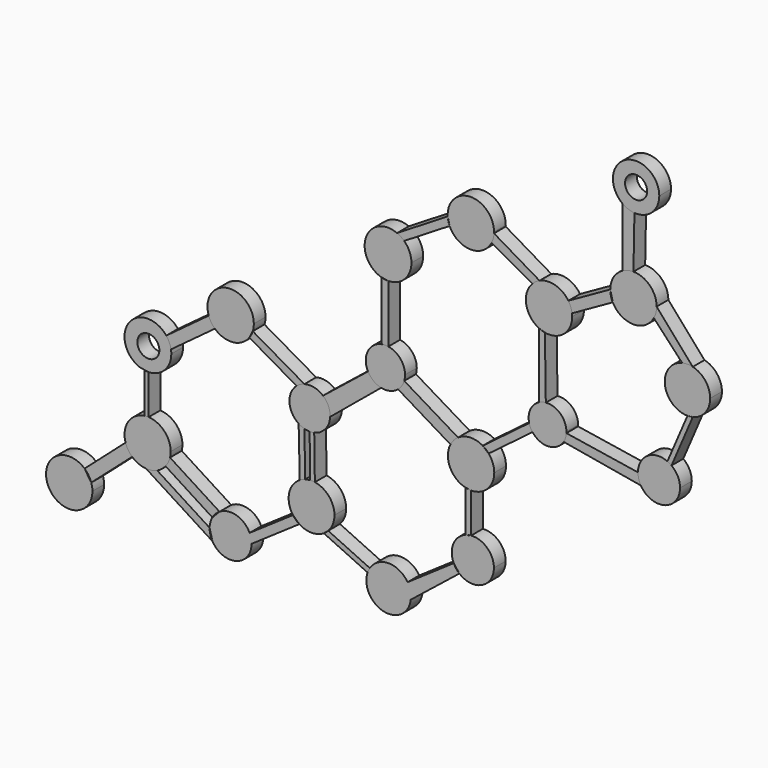
from build123d import *

# Parameters (mm, degrees)
F1_DEPTH = 2
F2_DEPTH = 2
F3_DEPTH = 2
F4_DEPTH = 2
F5_DEPTH = 2
F6_DEPTH = 2
F0_R     = 1.5066065713
F7_DEPTH = 2
F8_DEPTH = 2
F9_DEPTH = 2


# Not quite as in the source:
# - a feature names something its author has since deleted; it is built from what else it names


with BuildPart() as f1:
    # F0 (on Front) → F1 (new body)
    with BuildSketch(Plane.XZ):
        with BuildLine():
            ThreePointArc((-37.589425931, -3.0947996006), (-41.2739135306, 0.0261789427), (-43.7463731476, -4.1214588648))
            ThreePointArc((-43.7463731476, -4.1214588648), (-43.4052670506, -4.8209088), (-42.903755988, -5.4159468116))
            ThreePointArc((-42.903755988, -5.4159468116), (-40.446641178, -6.2439552219), (-38.1955916927, -4.9571812203))
            Line((-38.1955916927, -4.9571812203), (-37.7330076999, -4.0371317667))
            ThreePointArc((-37.7330076999, -4.0371317667), (-37.625527328, -3.5714036385), (-37.589425931, -3.0947996006))
        make_face()
        with BuildLine():
            Line((-43.7463731476, -4.1214588648), (-49.5391355238, -8.405172605))
            ThreePointArc((-49.5391355238, -8.405172605), (-49.1275958248, -9.0863151577), (-48.8971660779, -9.8480383571))
            Line((-48.8971660779, -9.8480383571), (-42.903755988, -5.4159468116))
            ThreePointArc((-42.903755988, -5.4159468116), (-43.4052670506, -4.8209088), (-43.7463731476, -4.1214588648))
        make_face()
    extrude(amount=F1_DEPTH)


with BuildPart() as f1b:
    # F0 (on Front) → F1, piece 2 (new body)
    with BuildSketch(Plane.XZ):
        with BuildLine():
            Line((-52.5149528088, -13.5454778642), (-52.5149528088, -19.0149929974))
            ThreePointArc((-52.5149528088, -19.0149929974), (-52.2351705303, -18.9893002665), (-51.9542118299, -18.9886305873))
            Line((-51.9542118299, -18.9886305873), (-51.9542118299, -13.5786520564))
            ThreePointArc((-51.9542118299, -13.5786520564), (-52.2353128072, -13.5744123442), (-52.5149528088, -13.5454778642))
        make_face()
    extrude(amount=F1_DEPTH)


with BuildPart() as f1c:
    # F0 (on Front) → F1, piece 3 (new body)
    with BuildSketch(Plane.XZ):
        with BuildLine():
            ThreePointArc((-60.6940817402, -28.0116869203), (-60.1449171731, -28.6432468808), (-59.7805504981, -29.396696701))
            Line((-59.7805504981, -29.396696701), (-54.1960356234, -24.4784262655))
            ThreePointArc((-54.1960356234, -24.4784262655), (-54.7415469087, -23.8352167765), (-55.0969163835, -23.0703549944))
            Line((-55.0969163835, -23.0703549944), (-60.6940817402, -28.0116869203))
        make_face()
    extrude(amount=F1_DEPTH)


with BuildPart() as f1d:
    # F0 (on Front) → F1, piece 4 (new body)
    with BuildSketch(Plane.XZ):
        with BuildLine():
            ThreePointArc((-60.6940817402, -28.0116869203), (-65.6698365107, -31.6876499309), (-59.622113901, -30.3853861988))
            ThreePointArc((-59.622113901, -30.3853861988), (-59.6619741252, -29.8847343541), (-59.7805504981, -29.396696701))
            Line((-59.7805504981, -29.396696701), (-60.6940817402, -28.0116869203))
        make_face()
    extrude(amount=F1_DEPTH)


with BuildPart() as f1e:
    # F0 (on Front) → F1, piece 5 (new body)
    with BuildSketch(Plane.XZ):
        with BuildLine():
            ThreePointArc((-49.0277410121, -22.8915968121), (-49.2667118253, -23.5421687766), (-49.6421238454, -24.124763615))
            Line((-49.6421238454, -24.124763615), (-43.2432128068, -28.2081848817))
            ThreePointArc((-43.2432128068, -28.2081848817), (-42.820009683, -27.6452432034), (-42.272247255, -27.2025688991))
            Line((-42.272247255, -27.2025688991), (-49.0277410121, -22.8915968121))
        make_face()
    extrude(amount=F1_DEPTH)


with BuildPart() as f1f:
    # F0 (on Front) → F1, piece 6 (new body)
    with BuildSketch(Plane.XZ):
        with BuildLine():
            ThreePointArc((-50.787159894, -25.0074364786), (-51.5279365519, -25.2380803723), (-52.3026155332, -25.2807317309))
            Line((-52.3026155332, -25.2807317309), (-43.2432128068, -31.0619275521))
            ThreePointArc((-43.2432128068, -31.0619275521), (-43.5341546393, -30.3463231537), (-43.623310519, -29.5789979072))
            Line((-43.623310519, -29.5789979072), (-50.787159894, -25.0074364786))
        make_face()
    extrude(amount=F1_DEPTH)


with BuildPart() as f1g:
    # F0 (on Front) → F1, piece 7 (new body)
    with BuildSketch(Plane.XZ):
        with BuildLine():
            ThreePointArc((-38.1675221321, -28.4145569119), (-37.9635998594, -29.0097260215), (-37.8945150633, -29.6350562169))
            Line((-37.8945150633, -29.6350562169), (-31.3852117273, -25.1609370351))
            ThreePointArc((-31.3852117273, -25.1609370351), (-31.85608698, -24.7950682197), (-32.2489724216, -24.3464876545))
            Line((-32.2489724216, -24.3464876545), (-38.1675221321, -28.4145569119))
        make_face()
        with BuildLine():
            Line((-43.623310519, -29.5789979072), (-43.2432128068, -31.0619275521))
            ThreePointArc((-43.2432128068, -31.0619275521), (-40.0208014314, -32.4029312754), (-37.8945150633, -29.6350562169))
            ThreePointArc((-37.8945150633, -29.6350562169), (-37.9635998594, -29.0097260215), (-38.1675221321, -28.4145569119))
            ThreePointArc((-38.1675221321, -28.4145569119), (-39.9479683628, -26.887644726), (-42.272247255, -27.2025688991))
            Line((-42.272247255, -27.2025688991), (-43.2432128068, -28.2081848817))
            ThreePointArc((-43.2432128068, -28.2081848817), (-43.5197045967, -28.8696225812), (-43.623310519, -29.5789979072))
        make_face()
    extrude(amount=F1_DEPTH)


with BuildPart() as f1h:
    # F0 (on Front) → F1, piece 8 (new body)
    with BuildSketch(Plane.XZ):
        with BuildLine():
            Line((-32.2489724216, -24.3464876545), (-31.3852117273, -25.1609370351))
            ThreePointArc((-31.3852117273, -25.1609370351), (-29.7102611512, -25.647195005), (-28.0353105751, -25.1609370351))
            Line((-28.0353105751, -25.1609370351), (-27.4344388987, -24.6650671828))
            ThreePointArc((-27.4344388987, -24.6650671828), (-26.8031946258, -23.6736847287), (-26.5823882584, -22.5193221122))
            ThreePointArc((-26.5823882584, -22.5193221122), (-27.3442929345, -20.4734034357), (-29.2588290055, -19.4241972599))
            ThreePointArc((-29.2588290055, -19.4241972599), (-29.5736466163, -19.3944340659), (-29.8898605352, -19.3966096864))
            ThreePointArc((-29.8898605352, -19.3966096864), (-30.2422535209, -19.4370221671), (-30.5878052461, -19.5170720902))
            ThreePointArc((-30.5878052461, -19.5170720902), (-30.9633331337, -19.6534192109), (-31.318418115, -19.8365213345))
            ThreePointArc((-31.318418115, -19.8365213345), (-32.7736054168, -21.8872534899), (-32.2489724216, -24.3464876545))
        make_face()
    extrude(amount=F1_DEPTH)


with BuildPart() as f1i:
    # F0 (on Front) → F1, piece 9 (new body)
    with BuildSketch(Plane.XZ):
        with BuildLine():
            ThreePointArc((-31.7558147602, -8.6673874945), (-32.7248214006, -10.9589087127), (-31.4725262417, -13.1087459619))
            ThreePointArc((-31.4725262417, -13.1087459619), (-31.0886843567, -13.3188508734), (-30.6766373042, -13.4661461312))
            ThreePointArc((-30.6766373042, -13.4661461312), (-30.3291581307, -13.5368601797), (-29.9755054116, -13.5627832774))
            ThreePointArc((-29.9755054116, -13.5627832774), (-29.6587887281, -13.5476755006), (-29.3458502966, -13.4966143551))
            ThreePointArc((-29.3458502966, -13.4966143551), (-28.9391104122, -13.3728908484), (-28.5559818149, -13.1886157349))
            Line((-28.5559818149, -13.1886157349), (-27.9344519304, -12.6986282105))
            ThreePointArc((-27.9344519304, -12.6986282105), (-27.3869776209, -11.8625662967), (-27.1704023319, -10.8869522401))
            ThreePointArc((-27.1704023319, -10.8869522401), (-27.1689132492, -10.8344270792), (-27.1684168293, -10.7818831599))
            ThreePointArc((-27.1684168293, -10.7818831599), (-27.4238049454, -9.6177281051), (-28.1430634561, -8.6673874945))
            ThreePointArc((-28.1430634561, -8.6673874945), (-29.3422205532, -8.0679615431), (-30.6824864397, -8.0992116323))
            ThreePointArc((-30.6824864397, -8.0992116323), (-31.2505437254, -8.3239955118), (-31.7558147602, -8.6673874945))
        make_face()
        with BuildLine():
            ThreePointArc((-37.7330076999, -4.0371317667), (-37.9266180846, -4.5161021168), (-38.1955916927, -4.9571812203))
            Line((-38.1955916927, -4.9571812203), (-31.7558147602, -8.6673874945))
            ThreePointArc((-31.7558147602, -8.6673874945), (-31.2505437254, -8.3239955118), (-30.6824864397, -8.0992116323))
            Line((-30.6824864397, -8.0992116323), (-37.7330076999, -4.0371317667))
        make_face()
        with BuildLine():
            Line((-22.0017600805, -3.7610865407), (-28.1430634561, -8.6673874945))
            ThreePointArc((-28.1430634561, -8.6673874945), (-27.4238049454, -9.6177281051), (-27.1684168293, -10.7818831599))
            ThreePointArc((-27.1684168293, -10.7818831599), (-27.1689132492, -10.8344270792), (-27.1704023319, -10.8869522401))
            Line((-27.1704023319, -10.8869522401), (-20.2051144084, -5.1334624074))
            ThreePointArc((-20.2051144084, -5.1334624074), (-21.2551436396, -4.6458808799), (-22.0017600805, -3.7610865407))
        make_face()
    extrude(amount=F1_DEPTH)


with BuildPart() as f1j:
    # F0 (on Front) → F1, piece 10 (new body)
    with BuildSketch(Plane.XZ):
        with BuildLine():
            ThreePointArc((-27.4344388987, -24.6650671828), (-27.7193761185, -24.931782603), (-28.0353105751, -25.1609370351))
            Line((-28.0353105751, -25.1609370351), (-22.0636666599, -27.9388750239))
            ThreePointArc((-22.0636666599, -27.9388750239), (-21.9298236713, -27.6131643375), (-21.7592310354, -27.3051066328))
            Line((-21.7592310354, -27.3051066328), (-27.4344388987, -24.6650671828))
        make_face()
    extrude(amount=F1_DEPTH)


with BuildPart() as f1k:
    # F0 (on Front) → F1, piece 11 (new body)
    with BuildSketch(Plane.XZ):
        with BuildLine():
            Line((-21.7592310354, -27.3051066328), (-22.0636666599, -27.9388750239))
            ThreePointArc((-22.0636666599, -27.9388750239), (-19.8661488676, -31.8951145091), (-16.1677066638, -29.2869656299))
            ThreePointArc((-16.1677066638, -29.2869656299), (-16.151956576, -29.1088509796), (-16.1467004913, -28.9301185889))
            ThreePointArc((-16.1467004913, -28.9301185889), (-16.2635315956, -28.0952311668), (-16.605049435, -27.324483426))
            ThreePointArc((-16.605049435, -27.324483426), (-19.1767786565, -25.8886276397), (-21.7592310354, -27.3051066328))
        make_face()
        with BuildLine():
            ThreePointArc((-16.1467004913, -28.9301185889), (-16.151956576, -29.1088509796), (-16.1677066638, -29.2869656299))
            Line((-16.1677066638, -29.2869656299), (-9.5345514551, -23.9877231505))
            ThreePointArc((-9.5345514551, -23.9877231505), (-9.97366221, -23.5326555023), (-10.3027902397, -22.9926744291))
            Line((-10.3027902397, -22.9926744291), (-16.605049435, -27.324483426))
            ThreePointArc((-16.605049435, -27.324483426), (-16.2635315956, -28.0952311668), (-16.1467004913, -28.9301185889))
        make_face()
    extrude(amount=F1_DEPTH)


with BuildPart() as f1l:
    # F0 (on Front) → F1, piece 12 (new body)
    with BuildSketch(Plane.XZ):
        with BuildLine():
            Line((-10.3027902397, -22.9926744291), (-9.5345514551, -23.9877231505))
            ThreePointArc((-9.5345514551, -23.9877231505), (-6.4727183358, -24.3792083426), (-4.8174418628, -21.7738019436))
            ThreePointArc((-4.8174418628, -21.7738019436), (-5.746709679, -19.6559016499), (-7.934436367, -18.9056401844))
            Line((-7.934436367, -18.9056401844), (-8.7257380015, -19.0864037696))
            ThreePointArc((-8.7257380015, -19.0864037696), (-10.3643389956, -20.6963441185), (-10.3027902397, -22.9926744291))
        make_face()
    extrude(amount=F1_DEPTH)


with BuildPart() as f1m:
    # F0 (on Front) → F1, piece 13 (new body)
    with BuildSketch(Plane.XZ):
        with BuildLine():
            Line((-8.7257380015, -13.3813622687), (-8.7257380015, -19.0864037696))
            ThreePointArc((-8.7257380015, -19.0864037696), (-8.3364915934, -18.9679863559), (-7.934436367, -18.9056401844))
            Line((-7.934436367, -18.9056401844), (-7.934436367, -13.4819080304))
            ThreePointArc((-7.934436367, -13.4819080304), (-8.3332683263, -13.4566709426), (-8.7257380015, -13.3813622687))
        make_face()
    extrude(amount=F1_DEPTH)


with BuildPart() as f1n:
    # F0 (on Front) → F1, piece 14 (new body)
    with BuildSketch(Plane.XZ):
        with BuildLine():
            ThreePointArc((-10.7471404399, -8.8686872464), (-10.8220432047, -11.6113089525), (-8.7257380015, -13.3813622687))
            Line((-8.7257380015, -13.3813622687), (-7.934436367, -13.4819080304))
            ThreePointArc((-7.934436367, -13.4819080304), (-5.6971007662, -12.555173281), (-4.7703660167, -10.3178376801))
            ThreePointArc((-4.7703660167, -10.3178376801), (-4.9665243966, -9.2210971833), (-5.5306776307, -8.2603428153))
            Line((-5.5306776307, -8.2603428153), (-6.3343212789, -7.5881906542))
            ThreePointArc((-6.3343212789, -7.5881906542), (-8.0398552645, -7.1555239643), (-9.7127880414, -7.7008152301))
            ThreePointArc((-9.7127880414, -7.7008152301), (-10.3030708851, -8.2200026768), (-10.7471404399, -8.8686872464))
        make_face()
    extrude(amount=F1_DEPTH)


with BuildPart() as f1o:
    # F0 (on Front) → F1, piece 15 (new body)
    with BuildSketch(Plane.XZ):
        with BuildLine():
            ThreePointArc((-6.3343212789, -7.5881906542), (-5.9044859902, -7.8907730644), (-5.5306776307, -8.2603428153))
            Line((-5.5306776307, -8.2603428153), (0.4520227905, -3.7452711915))
            ThreePointArc((0.4520227905, -3.7452711915), (0.1782258717, -3.2995528654), (0, -2.8077550232))
            Line((0, -2.8077550232), (-6.3343212789, -7.5881906542))
        make_face()
    extrude(amount=F1_DEPTH)


with BuildPart() as f1p:
    # F0 (on Front) → F1, piece 16 (new body)
    with BuildSketch(Plane.XZ):
        with BuildLine():
            Line((1.3706875539, 9.0120735989), (1.3706875539, 0.1384634004))
            ThreePointArc((1.3706875539, 0.1384634004), (1.8070578609, 0.3042996673), (2.2661741655, 0.3887563488))
            Line((2.2661741655, 0.3887563488), (2.1411547442, 8.7673323703))
            ThreePointArc((2.1411547442, 8.7673323703), (1.7480727228, 8.8649954394), (1.3706875539, 9.0120735989))
        make_face()
    extrude(amount=F1_DEPTH)


with BuildPart() as f1q:
    # F0 (on Front) → F1, piece 17 (new body)
    with BuildSketch(Plane.XZ):
        with BuildLine():
            ThreePointArc((0.4265353279, 14.0749963178), (-0.404465595, 11.3005324176), (1.3706875539, 9.0120735989))
            Line((1.3706875539, 9.0120735989), (2.1411547442, 8.7673323703))
            ThreePointArc((2.1411547442, 8.7673323703), (4.733812042, 9.4517433605), (5.8700526231, 11.8805800386))
            ThreePointArc((5.8700526231, 11.8805800386), (5.8634796502, 12.0844218734), (5.8437880405, 12.2874167948))
            ThreePointArc((5.8437880405, 12.2874167948), (5.6697146463, 12.9885654176), (5.3411360451, 13.6319525799))
            ThreePointArc((5.3411360451, 13.6319525799), (3.5849253378, 14.9201195219), (1.4122471164, 14.7680686579))
            ThreePointArc((1.4122471164, 14.7680686579), (0.8860935676, 14.46888958), (0.4265353279, 14.0749963178))
        make_face()
        with BuildLine():
            Line((11.0647150097, 16.8480308272), (5.3411360451, 13.6319525799))
            ThreePointArc((5.3411360451, 13.6319525799), (5.6697146463, 12.9885654176), (5.8437880405, 12.2874167948))
            Line((5.8437880405, 12.2874167948), (11.4082876159, 15.4141083547))
            ThreePointArc((11.4082876159, 15.4141083547), (11.1518067717, 16.1107764964), (11.0647150097, 16.8480308272))
        make_face()
    extrude(amount=F1_DEPTH)


with BuildPart() as f1r:
    # F0 (on Front) → F1, piece 18 (new body)
    with BuildSketch(Plane.XZ):
        with BuildLine():
            Line((-11.1217205665, 18.411016596), (-18.0350023015, 14.1660333875))
            ThreePointArc((-18.0350023015, 14.1660333875), (-17.5227173446, 13.8942737957), (-17.0679941499, 13.5343905243))
            Line((-17.0679941499, 13.5343905243), (-10.8623128482, 17.3448837072))
            ThreePointArc((-10.8623128482, 17.3448837072), (-11.0385836531, 17.8666196456), (-11.1217205665, 18.411016596))
        make_face()
        with BuildLine():
            Line((-20.166905726, 8.1530077233), (-19.2310512637, 8.0247410256))
            ThreePointArc((-19.2310512637, 8.0247410256), (-16.9970643361, 8.9740556334), (-16.074991523, 11.2194236533))
            ThreePointArc((-16.074991523, 11.2194236533), (-16.3337181015, 12.4789003135), (-17.0679941499, 13.5343905243))
            ThreePointArc((-17.0679941499, 13.5343905243), (-17.5227173446, 13.8942737957), (-18.0350023015, 14.1660333875))
            ThreePointArc((-18.0350023015, 14.1660333875), (-22.2811669762, 12.2870572206), (-20.166905726, 8.1530077233))
        make_face()
    extrude(amount=F1_DEPTH)


with BuildPart() as f1s:
    # F0 (on Front) → F1, piece 19 (new body)
    with BuildSketch(Plane.XZ):
        with BuildLine():
            Line((-20.166905726, 0.137046408), (-19.8017352531, 0.1608339565))
            ThreePointArc((-19.8017352531, 0.1608339565), (-19.5157580784, 0.1641787021), (-19.2310512637, 0.137046408))
            Line((-19.2310512637, 0.137046408), (-19.2310512637, 8.0247410256))
            ThreePointArc((-19.2310512637, 8.0247410256), (-19.7037450657, 8.0540967063), (-20.166905726, 8.1530077233))
            Line((-20.166905726, 8.1530077233), (-20.166905726, 0.137046408))
        make_face()
    extrude(amount=F1_DEPTH)


with BuildPart() as f1t:
    # F0 (on Front) → F1, piece 20 (new body)
    with BuildSketch(Plane.XZ):
        with BuildLine():
            Line((12.7010902051, 27.7389005383), (12.7010902051, 19.6188589877))
            ThreePointArc((12.7010902051, 19.6188589877), (13.4400376332, 19.9122139491), (14.22878536, 20.0121011774))
            Line((14.22878536, 20.0121011774), (14.3635529463, 27.1199137658))
            ThreePointArc((14.3635529463, 27.1199137658), (13.4880542027, 27.3105146948), (12.7010902051, 27.7389005383))
        make_face()
    extrude(amount=F1_DEPTH)


with BuildPart() as f1u:
    # F0 (on Front) → F1, piece 21 (new body)
    with BuildSketch(Plane.XZ):
        with BuildLine():
            Line((17.0147604727, 15.3481362132), (20.8823093018, 11.2153642881))
            ThreePointArc((20.8823093018, 11.2153642881), (21.6048193009, 11.3007129197), (22.3273293, 11.2153642881))
            Line((22.3273293, 11.2153642881), (17.3928557103, 16.8480308272))
            ThreePointArc((17.3928557103, 16.8480308272), (17.2968761696, 16.0746228071), (17.0147604727, 15.3481362132))
        make_face()
    extrude(amount=F1_DEPTH)


with BuildPart() as f1v:
    # F0 (on Front) → F1, piece 22 (new body)
    with BuildSketch(Plane.XZ):
        with BuildLine():
            Line((21.6048193009, 5.0990307341), (18.8674234688, -1.2655284067))
            ThreePointArc((18.8674234688, -1.2655284067), (19.1558508738, -1.4112828883), (19.4260827802, -1.5885100127))
            Line((19.4260827802, -1.5885100127), (22.3273293, 5.1843793656))
            ThreePointArc((22.3273293, 5.1843793656), (21.9685860832, 5.1204418129), (21.6048193009, 5.0990307341))
        make_face()
    extrude(amount=F1_DEPTH)


with BuildPart() as f1w:
    # F0 (on Front) → F1, piece 23 (new body)
    with BuildSketch(Plane.XZ):
        with BuildLine():
            ThreePointArc((5.073574541, -2.3652681739), (4.9561703, -2.9698845171), (4.6987535943, -3.5294212164))
            Line((4.6987535943, -3.5294212164), (15.2385687415, -5.3491116368))
            ThreePointArc((15.2385687415, -5.3491116368), (14.9453544153, -4.6498799144), (14.8452927694, -3.8982900596))
            Line((14.8452927694, -3.8982900596), (5.073574541, -2.3652681739))
        make_face()
    extrude(amount=F1_DEPTH)


with BuildPart() as f2:
    # F0 (on Front) → F2 (new body)
    with BuildSketch(Plane.XZ):
        with BuildLine():
            Line((-17.9006594395, -4.5664300135), (-10.7471404399, -8.8686872464))
            ThreePointArc((-10.7471404399, -8.8686872464), (-10.3030708851, -8.2200026768), (-9.7127880414, -7.7008152301))
            Line((-9.7127880414, -7.7008152301), (-17.0583318909, -3.2830707385))
            ThreePointArc((-17.0583318909, -3.2830707385), (-17.3856953146, -3.9863158479), (-17.9006594395, -4.5664300135))
        make_face()
    extrude(amount=F2_DEPTH)


with BuildPart() as f3:
    # F0 (on Front) → F3 (new body)
    with BuildSketch(Plane.XZ):
        with BuildLine():
            Line((-22.0017600805, -3.7610865407), (-28.1430634561, -8.6673874945))
            ThreePointArc((-28.1430634561, -8.6673874945), (-27.4238049454, -9.6177281051), (-27.1684168293, -10.7818831599))
            ThreePointArc((-27.1684168293, -10.7818831599), (-27.1689132492, -10.8344270792), (-27.1704023319, -10.8869522401))
            Line((-27.1704023319, -10.8869522401), (-20.2051144084, -5.1334624074))
            ThreePointArc((-20.2051144084, -5.1334624074), (-21.2551436396, -4.6458808799), (-22.0017600805, -3.7610865407))
        make_face()
    extrude(amount=F3_DEPTH)


with BuildPart() as f4:
    # F0 (on Front) → F4 (new body)
    with BuildSketch(Plane.XZ):
        with BuildLine():
            Line((-31.4725262417, -13.1087459619), (-31.318418115, -19.8365213345))
            ThreePointArc((-31.318418115, -19.8365213345), (-30.9633331337, -19.6534192109), (-30.5878052461, -19.5170720902))
            Line((-30.5878052461, -19.5170720902), (-30.6766373042, -13.4661461312))
            ThreePointArc((-30.6766373042, -13.4661461312), (-31.0886843567, -13.3188508734), (-31.4725262417, -13.1087459619))
        make_face()
    extrude(amount=F4_DEPTH)


with BuildPart() as f5:
    # F0 (on Front) → F5 (new body)
    with BuildSketch(Plane.XZ):
        with BuildLine():
            Line((-22.0017600805, -3.7610865407), (-28.1430634561, -8.6673874945))
            ThreePointArc((-28.1430634561, -8.6673874945), (-27.4238049454, -9.6177281051), (-27.1684168293, -10.7818831599))
            ThreePointArc((-27.1684168293, -10.7818831599), (-27.1689132492, -10.8344270792), (-27.1704023319, -10.8869522401))
            Line((-27.1704023319, -10.8869522401), (-20.2051144084, -5.1334624074))
            ThreePointArc((-20.2051144084, -5.1334624074), (-21.2551436396, -4.6458808799), (-22.0017600805, -3.7610865407))
        make_face()
    extrude(amount=F5_DEPTH)


with BuildPart() as f5b:
    # F0 (on Front) → F5, piece 2 (new body)
    with BuildSketch(Plane.XZ):
        with BuildLine():
            Line((-29.9755054116, -13.5627832774), (-29.8898605352, -19.3966096864))
            ThreePointArc((-29.8898605352, -19.3966096864), (-29.5736466163, -19.3944340659), (-29.2588290055, -19.4241972599))
            Line((-29.2588290055, -19.4241972599), (-29.3458502966, -13.4966143551))
            ThreePointArc((-29.3458502966, -13.4966143551), (-29.6587887281, -13.5476755006), (-29.9755054116, -13.5627832774))
        make_face()
    extrude(amount=F5_DEPTH)


with BuildPart() as f6:
    # F0 (on Front) → F6 (new body)
    with BuildSketch(Plane.XZ):
        with BuildLine():
            ThreePointArc((-37.589425931, -3.0947996006), (-41.2739135306, 0.0261789427), (-43.7463731476, -4.1214588648))
            ThreePointArc((-43.7463731476, -4.1214588648), (-43.4052670506, -4.8209088), (-42.903755988, -5.4159468116))
            ThreePointArc((-42.903755988, -5.4159468116), (-40.446641178, -6.2439552219), (-38.1955916927, -4.9571812203))
            Line((-38.1955916927, -4.9571812203), (-37.7330076999, -4.0371317667))
            ThreePointArc((-37.7330076999, -4.0371317667), (-37.625527328, -3.5714036385), (-37.589425931, -3.0947996006))
        make_face()
    extrude(amount=F6_DEPTH)


with BuildPart() as f6b:
    # F0 (on Front) → F6, piece 2 (new body)
    with BuildSketch(Plane.XZ):
        with BuildLine():
            Line((-52.5149528088, -13.4941877539), (-51.9542118299, -13.5786520564))
            ThreePointArc((-51.9542118299, -13.5786520564), (-49.7550373735, -12.6113053664), (-48.8517080577, -10.3850699666))
            ThreePointArc((-48.8517080577, -10.3850699666), (-48.863092847, -10.1155939096), (-48.8971660779, -9.8480383571))
            ThreePointArc((-48.8971660779, -9.8480383571), (-49.1275958248, -9.0863151577), (-49.5391355238, -8.405172605))
            ThreePointArc((-49.5391355238, -8.405172605), (-54.6558064246, -8.5412451571), (-53.0756937878, -13.4097234514))
            Line((-53.0756937878, -13.4097234514), (-52.5149528088, -13.4941877539))
        make_face()
        with Locations((-51.9861578941, -10.463591665)):
            Circle(F0_R, mode=Mode.SUBTRACT)
    extrude(amount=F6_DEPTH)


with BuildPart() as f6c:
    # F0 (on Front) → F6, piece 3 (new body)
    with BuildSketch(Plane.XZ):
        with BuildLine():
            ThreePointArc((-31.7558147602, -8.6673874945), (-32.7248214006, -10.9589087127), (-31.4725262417, -13.1087459619))
            ThreePointArc((-31.4725262417, -13.1087459619), (-31.0886843567, -13.3188508734), (-30.6766373042, -13.4661461312))
            ThreePointArc((-30.6766373042, -13.4661461312), (-30.3291581307, -13.5368601797), (-29.9755054116, -13.5627832774))
            ThreePointArc((-29.9755054116, -13.5627832774), (-29.6587887281, -13.5476755006), (-29.3458502966, -13.4966143551))
            ThreePointArc((-29.3458502966, -13.4966143551), (-28.9391104122, -13.3728908484), (-28.5559818149, -13.1886157349))
            Line((-28.5559818149, -13.1886157349), (-27.9344519304, -12.6986282105))
            ThreePointArc((-27.9344519304, -12.6986282105), (-27.3869776209, -11.8625662967), (-27.1704023319, -10.8869522401))
            ThreePointArc((-27.1704023319, -10.8869522401), (-27.1689132492, -10.8344270792), (-27.1684168293, -10.7818831599))
            ThreePointArc((-27.1684168293, -10.7818831599), (-27.4238049454, -9.6177281051), (-28.1430634561, -8.6673874945))
            ThreePointArc((-28.1430634561, -8.6673874945), (-29.3422205532, -8.0679615431), (-30.6824864397, -8.0992116323))
            ThreePointArc((-30.6824864397, -8.0992116323), (-31.2505437254, -8.3239955118), (-31.7558147602, -8.6673874945))
        make_face()
        with BuildLine():
            Line((-22.0017600805, -3.7610865407), (-28.1430634561, -8.6673874945))
            ThreePointArc((-28.1430634561, -8.6673874945), (-27.4238049454, -9.6177281051), (-27.1684168293, -10.7818831599))
            ThreePointArc((-27.1684168293, -10.7818831599), (-27.1689132492, -10.8344270792), (-27.1704023319, -10.8869522401))
            Line((-27.1704023319, -10.8869522401), (-20.2051144084, -5.1334624074))
            ThreePointArc((-20.2051144084, -5.1334624074), (-21.2551436396, -4.6458808799), (-22.0017600805, -3.7610865407))
        make_face()
    extrude(amount=F6_DEPTH)


with BuildPart() as f6d:
    # F0 (on Front) → F6, piece 4 (new body)
    with BuildSketch(Plane.XZ):
        with BuildLine():
            Line((-20.166905726, 8.1530077233), (-19.2310512637, 8.0247410256))
            ThreePointArc((-19.2310512637, 8.0247410256), (-16.9970643361, 8.9740556334), (-16.074991523, 11.2194236533))
            ThreePointArc((-16.074991523, 11.2194236533), (-16.3337181015, 12.4789003135), (-17.0679941499, 13.5343905243))
            ThreePointArc((-17.0679941499, 13.5343905243), (-17.5227173446, 13.8942737957), (-18.0350023015, 14.1660333875))
            ThreePointArc((-18.0350023015, 14.1660333875), (-22.2811669762, 12.2870572206), (-20.166905726, 8.1530077233))
        make_face()
    extrude(amount=F6_DEPTH)


with BuildPart() as f6e:
    # F0 (on Front) → F6, piece 5 (new body)
    with BuildSketch(Plane.XZ):
        with BuildLine():
            ThreePointArc((-4.8001403762, 18.614665292), (-8.0660878972, 21.7770950894), (-11.1217205665, 18.411016596))
            Line((-11.1217205665, 18.411016596), (-10.8623128482, 17.3448837072))
            ThreePointArc((-10.8623128482, 17.3448837072), (-8.0490426257, 15.4517323603), (-5.1383388486, 17.1913630363))
            ThreePointArc((-5.1383388486, 17.1913630363), (-4.9083346697, 17.7943222496), (-4.8054518647, 18.4314069094))
            ThreePointArc((-4.8054518647, 18.4314069094), (-4.8014685271, 18.5229976223), (-4.8001403762, 18.614665292))
        make_face()
    extrude(amount=F6_DEPTH)


with BuildPart() as f6f:
    # F0 (on Front) → F6, piece 6 (new body)
    with BuildSketch(Plane.XZ):
        with BuildLine():
            ThreePointArc((0, -2.8077550232), (0.1782258717, -3.2995528654), (0.4520227905, -3.7452711915))
            ThreePointArc((0.4520227905, -3.7452711915), (2.6322031678, -4.7551499279), (4.6987535943, -3.5294212164))
            ThreePointArc((4.6987535943, -3.5294212164), (4.9561703, -2.9698845171), (5.073574541, -2.3652681739))
            ThreePointArc((5.073574541, -2.3652681739), (5.07859903, -2.2724391904), (5.0802745854, -2.1794894287))
            ThreePointArc((5.0802745854, -2.1794894287), (4.2397953639, -0.2745584885), (2.2661741655, 0.3887563488))
            ThreePointArc((2.2661741655, 0.3887563488), (1.8070578609, 0.3042996673), (1.3706875539, 0.1384634004))
            ThreePointArc((1.3706875539, 0.1384634004), (0.1629760262, -1.0916214081), (0, -2.8077550232))
        make_face()
    extrude(amount=F6_DEPTH)


with BuildPart() as f6g:
    # F0 (on Front) → F6, piece 7 (new body)
    with BuildSketch(Plane.XZ):
        with BuildLine():
            ThreePointArc((0.4265353279, 14.0749963178), (-0.404465595, 11.3005324176), (1.3706875539, 9.0120735989))
            Line((1.3706875539, 9.0120735989), (2.1411547442, 8.7673323703))
            ThreePointArc((2.1411547442, 8.7673323703), (4.733812042, 9.4517433605), (5.8700526231, 11.8805800386))
            ThreePointArc((5.8700526231, 11.8805800386), (5.8634796502, 12.0844218734), (5.8437880405, 12.2874167948))
            ThreePointArc((5.8437880405, 12.2874167948), (5.6697146463, 12.9885654176), (5.3411360451, 13.6319525799))
            ThreePointArc((5.3411360451, 13.6319525799), (3.5849253378, 14.9201195219), (1.4122471164, 14.7680686579))
            ThreePointArc((1.4122471164, 14.7680686579), (0.8860935676, 14.46888958), (0.4265353279, 14.0749963178))
        make_face()
    extrude(amount=F6_DEPTH)


with BuildPart() as f7:
    # F0 (on Front) → F7 (new body)
    with BuildSketch(Plane.XZ):
        with BuildLine():
            ThreePointArc((-55.0969163835, -23.0703549944), (-54.7415469087, -23.8352167765), (-54.1960356234, -24.4784262655))
            ThreePointArc((-54.1960356234, -24.4784262655), (-53.316613571, -25.0383769157), (-52.3026155332, -25.2807317309))
            ThreePointArc((-52.3026155332, -25.2807317309), (-51.5279365519, -25.2380803723), (-50.787159894, -25.0074364786))
            ThreePointArc((-50.787159894, -25.0074364786), (-50.1633359059, -24.6326560502), (-49.6421238454, -24.124763615))
            ThreePointArc((-49.6421238454, -24.124763615), (-49.2667118253, -23.5421687766), (-49.0277410121, -22.8915968121))
            ThreePointArc((-49.0277410121, -22.8915968121), (-48.9590548353, -22.5170555161), (-48.936047454, -22.1369639039))
            ThreePointArc((-48.936047454, -22.1369639039), (-49.8124667832, -19.9562920537), (-51.9542118299, -18.9886305873))
            ThreePointArc((-51.9542118299, -18.9886305873), (-52.2351705303, -18.9893002665), (-52.5149528088, -19.0149929974))
            ThreePointArc((-52.5149528088, -19.0149929974), (-54.7453038093, -20.4445974016), (-55.0969163835, -23.0703549944))
        make_face()
    extrude(amount=F7_DEPTH)


with BuildPart() as f7b:
    # F0 (on Front) → F7, piece 2 (new body)
    with BuildSketch(Plane.XZ):
        with BuildLine():
            ThreePointArc((-31.7558147602, -8.6673874945), (-32.7248214006, -10.9589087127), (-31.4725262417, -13.1087459619))
            ThreePointArc((-31.4725262417, -13.1087459619), (-31.0886843567, -13.3188508734), (-30.6766373042, -13.4661461312))
            ThreePointArc((-30.6766373042, -13.4661461312), (-30.3291581307, -13.5368601797), (-29.9755054116, -13.5627832774))
            ThreePointArc((-29.9755054116, -13.5627832774), (-29.6587887281, -13.5476755006), (-29.3458502966, -13.4966143551))
            ThreePointArc((-29.3458502966, -13.4966143551), (-28.9391104122, -13.3728908484), (-28.5559818149, -13.1886157349))
            Line((-28.5559818149, -13.1886157349), (-27.9344519304, -12.6986282105))
            ThreePointArc((-27.9344519304, -12.6986282105), (-27.3869776209, -11.8625662967), (-27.1704023319, -10.8869522401))
            ThreePointArc((-27.1704023319, -10.8869522401), (-27.1689132492, -10.8344270792), (-27.1684168293, -10.7818831599))
            ThreePointArc((-27.1684168293, -10.7818831599), (-27.4238049454, -9.6177281051), (-28.1430634561, -8.6673874945))
            ThreePointArc((-28.1430634561, -8.6673874945), (-29.3422205532, -8.0679615431), (-30.6824864397, -8.0992116323))
            ThreePointArc((-30.6824864397, -8.0992116323), (-31.2505437254, -8.3239955118), (-31.7558147602, -8.6673874945))
        make_face()
    extrude(amount=F7_DEPTH)


with BuildPart() as f7c:
    # F0 (on Front) → F7, piece 3 (new body)
    with BuildSketch(Plane.XZ):
        with BuildLine():
            ThreePointArc((0, -2.8077550232), (0.1782258717, -3.2995528654), (0.4520227905, -3.7452711915))
            ThreePointArc((0.4520227905, -3.7452711915), (2.6322031678, -4.7551499279), (4.6987535943, -3.5294212164))
            ThreePointArc((4.6987535943, -3.5294212164), (4.9561703, -2.9698845171), (5.073574541, -2.3652681739))
            ThreePointArc((5.073574541, -2.3652681739), (5.07859903, -2.2724391904), (5.0802745854, -2.1794894287))
            ThreePointArc((5.0802745854, -2.1794894287), (4.2397953639, -0.2745584885), (2.2661741655, 0.3887563488))
            ThreePointArc((2.2661741655, 0.3887563488), (1.8070578609, 0.3042996673), (1.3706875539, 0.1384634004))
            ThreePointArc((1.3706875539, 0.1384634004), (0.1629760262, -1.0916214081), (0, -2.8077550232))
        make_face()
    extrude(amount=F7_DEPTH)


with BuildPart() as f7d:
    # F0 (on Front) → F7, piece 4 (new body)
    with BuildSketch(Plane.XZ):
        with BuildLine():
            ThreePointArc((14.8452927694, -3.8982900596), (14.9453544153, -4.6498799144), (15.2385687415, -5.3491116368))
            ThreePointArc((15.2385687415, -5.3491116368), (18.4696099186, -6.6709557082), (20.5907473583, -3.8982900596))
            ThreePointArc((20.5907473583, -3.8982900596), (20.2831088044, -2.6048907164), (19.4260827802, -1.5885100127))
            ThreePointArc((19.4260827802, -1.5885100127), (19.1558508738, -1.4112828883), (18.8674234688, -1.2655284067))
            ThreePointArc((18.8674234688, -1.2655284067), (16.1447051598, -1.4947005936), (14.8452927694, -3.8982900596))
        make_face()
    extrude(amount=F7_DEPTH)


with BuildPart() as f7e:
    # F0 (on Front) → F7, piece 5 (new body)
    with BuildSketch(Plane.XZ):
        with BuildLine():
            ThreePointArc((20.8823093018, 11.2153642881), (18.5253892869, 7.8361050445), (21.6048193009, 5.0990307341))
            Line((21.6048193009, 5.0990307341), (22.3273293, 5.1843793656))
            ThreePointArc((22.3273293, 5.1843793656), (24.0395271045, 6.2796079404), (24.7056603937, 8.1998718269))
            ThreePointArc((24.7056603937, 8.1998718269), (24.0395271045, 10.1201357134), (22.3273293, 11.2153642881))
            ThreePointArc((22.3273293, 11.2153642881), (21.6048193009, 11.3007129197), (20.8823093018, 11.2153642881))
        make_face()
    extrude(amount=F7_DEPTH)


with BuildPart() as f7f:
    # F0 (on Front) → F7, piece 6 (new body)
    with BuildSketch(Plane.XZ):
        with BuildLine():
            ThreePointArc((12.7010902051, 19.6188589877), (11.5043518294, 18.4570066252), (11.0647150097, 16.8480308272))
            Line((11.0647150097, 16.8480308272), (11.4082876159, 15.4141083547))
            ThreePointArc((11.4082876159, 15.4141083547), (14.191555884, 13.6841795115), (17.0147604727, 15.3481362132))
            ThreePointArc((17.0147604727, 15.3481362132), (17.2968761696, 16.0746228071), (17.3928557103, 16.8480308272))
            ThreePointArc((17.3928557103, 16.8480308272), (16.4661209608, 19.085366428), (14.22878536, 20.0121011774))
            ThreePointArc((14.22878536, 20.0121011774), (13.4400376332, 19.9122139491), (12.7010902051, 19.6188589877))
        make_face()
    extrude(amount=F7_DEPTH)


with BuildPart() as f7g:
    # F0 (on Front) → F7, piece 7 (new body)
    with BuildSketch(Plane.XZ):
        with BuildLine():
            ThreePointArc((17.7561629195, 30.2757196568), (13.1729243852, 33.1036699476), (12.7010902051, 27.7389005383))
            ThreePointArc((12.7010902051, 27.7389005383), (13.4880542027, 27.3105146948), (14.3635529463, 27.1199137658))
            ThreePointArc((14.3635529463, 27.1199137658), (16.7471129562, 27.9589917244), (17.7561629195, 30.2757196568))
        make_face()
        with Locations((14.5920925692, 30.2757196568)):
            Circle(F0_R, mode=Mode.SUBTRACT)
    extrude(amount=F7_DEPTH)


with BuildPart() as f7h:
    # F0 (on Front) → F7, piece 8 (new body)
    with BuildSketch(Plane.XZ):
        with BuildLine():
            ThreePointArc((0.4265353279, 14.0749963178), (-0.404465595, 11.3005324176), (1.3706875539, 9.0120735989))
            Line((1.3706875539, 9.0120735989), (2.1411547442, 8.7673323703))
            ThreePointArc((2.1411547442, 8.7673323703), (4.733812042, 9.4517433605), (5.8700526231, 11.8805800386))
            ThreePointArc((5.8700526231, 11.8805800386), (5.8634796502, 12.0844218734), (5.8437880405, 12.2874167948))
            ThreePointArc((5.8437880405, 12.2874167948), (5.6697146463, 12.9885654176), (5.3411360451, 13.6319525799))
            ThreePointArc((5.3411360451, 13.6319525799), (3.5849253378, 14.9201195219), (1.4122471164, 14.7680686579))
            ThreePointArc((1.4122471164, 14.7680686579), (0.8860935676, 14.46888958), (0.4265353279, 14.0749963178))
        make_face()
    extrude(amount=F7_DEPTH)


with BuildPart() as f8:
    # F0 (on Front) → F8 (new body)
    with BuildSketch(Plane.XZ):
        with BuildLine():
            ThreePointArc((-19.8017352531, 0.1608339565), (-21.9660735403, -1.2030863093), (-22.0017600805, -3.7610865407))
            ThreePointArc((-22.0017600805, -3.7610865407), (-21.2551436396, -4.6458808799), (-20.2051144084, -5.1334624074))
            ThreePointArc((-20.2051144084, -5.1334624074), (-18.9867420931, -5.1187629229), (-17.9006594395, -4.5664300135))
            ThreePointArc((-17.9006594395, -4.5664300135), (-17.3856953146, -3.9863158479), (-17.0583318909, -3.2830707385))
            ThreePointArc((-17.0583318909, -3.2830707385), (-16.9742051796, -2.9031040055), (-16.9459646612, -2.5149616413))
            ThreePointArc((-16.9459646612, -2.5149616413), (-17.596034833, -0.7646211405), (-19.2310512637, 0.137046408))
            ThreePointArc((-19.2310512637, 0.137046408), (-19.5157580784, 0.1641787021), (-19.8017352531, 0.1608339565))
        make_face()
    extrude(amount=F8_DEPTH)


with BuildPart() as f8b:
    # F0 (on Front) → F8, piece 2 (new body)
    with BuildSketch(Plane.XZ):
        with BuildLine():
            ThreePointArc((-4.8054518647, 18.4314069094), (-4.9083346697, 17.7943222496), (-5.1383388486, 17.1913630363))
            Line((-5.1383388486, 17.1913630363), (0.4265353279, 14.0749963178))
            ThreePointArc((0.4265353279, 14.0749963178), (0.8860935676, 14.46888958), (1.4122471164, 14.7680686579))
            Line((1.4122471164, 14.7680686579), (-4.8054518647, 18.4314069094))
        make_face()
    extrude(amount=F8_DEPTH)


with BuildPart() as f9:
    # F0 (on Front) → F9 (new body)
    with BuildSketch(Plane.XZ):
        with BuildLine():
            Line((-43.7463731476, -4.1214588648), (-49.5391355238, -8.405172605))
            ThreePointArc((-49.5391355238, -8.405172605), (-49.1275958248, -9.0863151577), (-48.8971660779, -9.8480383571))
            Line((-48.8971660779, -9.8480383571), (-42.903755988, -5.4159468116))
            ThreePointArc((-42.903755988, -5.4159468116), (-43.4052670506, -4.8209088), (-43.7463731476, -4.1214588648))
        make_face()
    extrude(amount=F9_DEPTH)


solid = Compound([f1.part, f1b.part, f1c.part, f1d.part, f1e.part, f1f.part, f1g.part, f1h.part, f1i.part, f1j.part, f1k.part, f1l.part, f1m.part, f1n.part, f1o.part, f1p.part, f1q.part, f1r.part, f1s.part, f1t.part, f1u.part, f1v.part, f1w.part, f2.part, f3.part, f4.part, f5.part, f5b.part, f6.part, f6b.part, f6c.part, f6d.part, f6e.part, f6f.part, f6g.part, f7.part, f7b.part, f7c.part, f7d.part, f7e.part, f7f.part, f7g.part, f7h.part, f8.part, f8b.part, f9.part])
